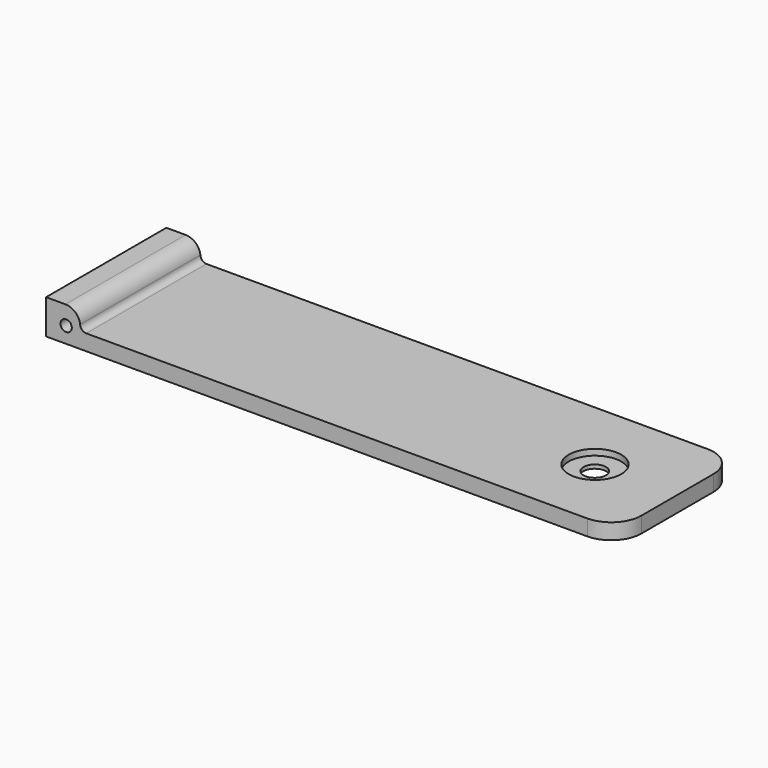
from build123d import *

# Parameters (mm, degrees)
F1_DEPTH  = 2.1
F2_R      = 1.5
F3_DEPTH  = 2.101
F5_DEPTH  = 0.8
F6_R      = 4.5
F6_R_2    = 1.5
F7_DEPTH  = 0.8
F9_DEPTH  = 20
F10_R     = 0.75
F11_DEPTH = 20.001


# Not quite as in the source:
# - a feature names something its author has since deleted; it is built from what else it names


with BuildPart() as f1:
    # F0 (on Top) → F1 (new body)
    with BuildSketch(Plane.XY):
        with BuildLine():
            Line((-61.724215433, 4.4804378226), (-61.724215433, -15.5195621774))
            Line((-61.724215433, -15.5195621774), (10.275784567, -15.5195621774))
            ThreePointArc((10.275784567, -15.5195621774), (13.1042116917, -14.3479893021), (14.275784567, -11.5195621774))
            Line((14.275784567, -11.5195621774), (14.275784567, -5.5195621774))
            Line((14.275784567, -5.5195621774), (14.275784567, 0.4804378226))
            ThreePointArc((14.275784567, 0.4804378226), (13.1042116917, 3.3088649474), (10.275784567, 4.4804378226))
            Line((10.275784567, 4.4804378226), (-61.724215433, 4.4804378226))
        make_face()
    extrude(amount=-F1_DEPTH)

    # F2 (on face) → F3 (cut, through all)
    with BuildSketch(Plane(origin=(0, 0, -2.1), x_dir=(1, 0, 0), z_dir=(0, 0, -1))):
        with Locations((3.2757834997, 5.5195621774)):
            Circle(F2_R)
    extrude(amount=-F3_DEPTH, mode=Mode.SUBTRACT)

    # F4 (on face) → F5 (cut)
    with BuildSketch(Plane.XY):
        with BuildLine():
            ThreePointArc((6.808292926, -5.5195621774), (-0.1917041784, -5.5256023727), (6.8082952425, -5.523588974))
            ThreePointArc((6.8082952425, -5.523588974), (6.8082946634, -5.5215755754), (6.808292926, -5.5195621774))
        make_face()
    extrude(amount=-F5_DEPTH, mode=Mode.SUBTRACT)

    # F6 (on face) → F7 (cut)
    with BuildSketch(Plane(origin=(0, 0, -2.1), x_dir=(1, 0, 0), z_dir=(0, 0, -1))):
        with Locations((3.2757834997, 5.5195621774)):
            Circle(F6_R)
        with Locations((3.2757834997, 5.5195621774)):
            Circle(F6_R_2, mode=Mode.SUBTRACT)
    extrude(amount=-F7_DEPTH, mode=Mode.SUBTRACT)

    # F8 (on face) → F9 (join)
    with BuildSketch(Plane.XZ.offset(15.5195621774)):
        with BuildLine():
            Line((-59.1665172217, 2.5), (-61.724215433, 2.5))
            Line((-61.724215433, 2.5), (-61.724215433, 0))
            Line((-61.724215433, 0), (-57.1891452284, 0))
            Line((-57.1891452284, 0), (-56.3891452284, 0))
            ThreePointArc((-56.3891452284, 0), (-56.9548306533, 0.2343145751), (-57.1891452284, 0.8))
            ThreePointArc((-57.1891452284, 0.8), (-57.8626767407, 2.0165750888), (-59.1665172217, 2.5))
        make_face()
    extrude(amount=-F9_DEPTH)

    # F10 (on face) → F11 (cut, through all)
    with BuildSketch(Plane(origin=(0, 4.4804378226, 0), x_dir=(-1, 0, 0), z_dir=(0, 1, 0))):
        with Locations((59.05039973, 0.0338958319)):
            Circle(F10_R)
    extrude(amount=-F11_DEPTH, mode=Mode.SUBTRACT)


solid = f1.part
